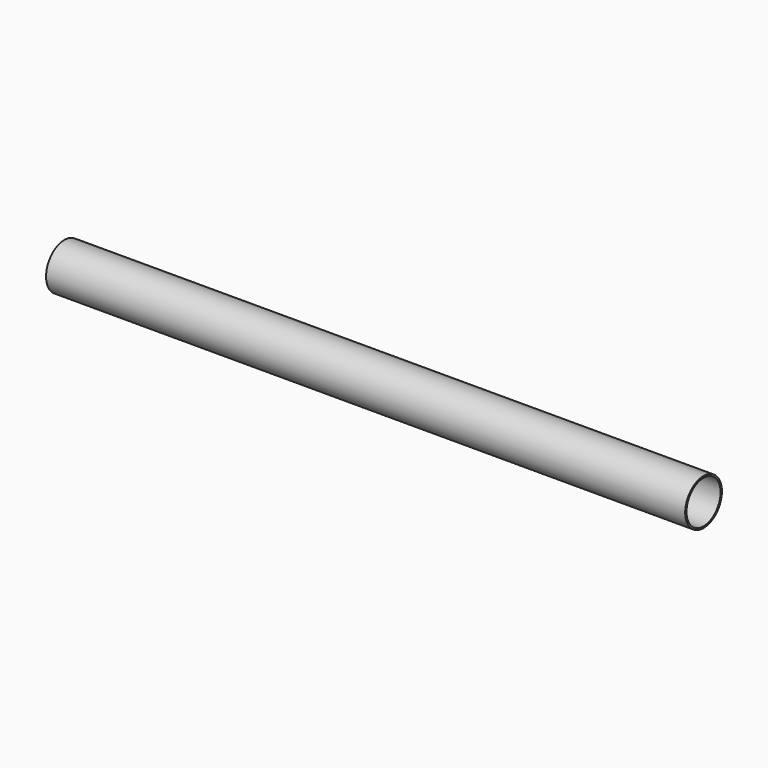
from build123d import *

# Parameters (mm, degrees)
F1_R     = 109.5375
F1_R_2   = 101.6
F2_DEPTH = 3048


# Not quite as in the source:
# - a variable given as a bare number and used for a length is read in inches; the dataset says mm whatever the document's units were


with BuildPart() as f2:
    # F1 (on Right) → F2 (new body)
    with BuildSketch(Plane.YZ):
        Circle(F1_R)
        Circle(F1_R_2, mode=Mode.SUBTRACT)
    extrude(amount=-F2_DEPTH)


solid = f2.part
